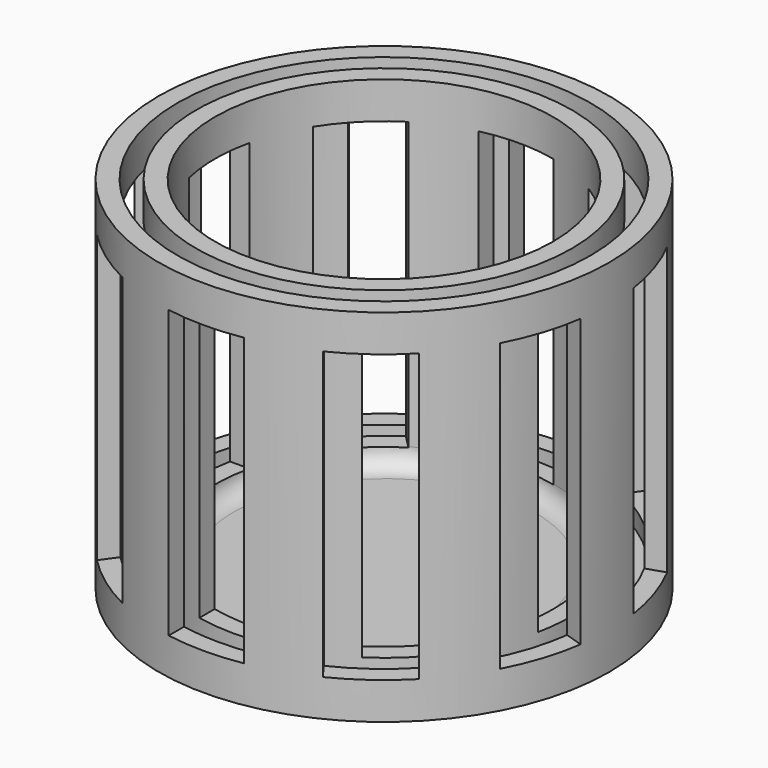
from build123d import *

# Parameters (mm, degrees)
F2_W            = 20
F2_H            = 76.3443418741
F3_REACH        = 138.9215837294
F3_COPIES_COUNT = 8
F5_W            = 20
F5_H            = 76.3443418741
F6_REACH        = 213.9215837294
F6_COPIES_COUNT = 10


# Not quite as in the source:
# - a pattern or mirror of a feature is missing from the dataset's text; its kind, count and spacing are read off the source's solid


with BuildPart() as f1:
    # F0 (on Front) → F1 (revolve)
    with BuildSketch(Plane.XZ):
        with BuildLine():
            Line((0, 5), (0, 0))
            Line((0, 0), (60, 0))
            Line((60, 0), (60, 96))
            Line((60, 96), (55, 96))
            Line((55, 96), (55, 5))
            Line((55, 5), (50, 5))
            Line((50, 5), (50, 96))
            Line((50, 96), (45, 96))
            Line((45, 96), (45, 10))
            ThreePointArc((45, 10), (43.5355339059, 6.4644660941), (40, 5))
            Line((40, 5), (0, 5))
        make_face()
    revolve(axis=Axis((0, 0, 2.5), (0, 0, 1)))

    f3_end = f1.faces().sort_by_distance((-50, 0, 50.5))[0]
    # F2 (on Front) → F3 (cut, up to a face of the model that its end follows)
    with BuildSketch(Plane.XZ):
        with Locations((0, 48)):
            Rectangle(F2_W, F2_H)
    f3_long = extrude(amount=F3_REACH, mode=Mode.PRIVATE)
    f3 = split(f3_long, bisect_by=f3_end, keep=Keep.BOTTOM, mode=Mode.PRIVATE)
    add(f3, mode=Mode.SUBTRACT)

    # F3_copies: F3 ×8 about axis
    f3_copies_axis = Axis((0, 0, 0), (0, 0, 1))
    for i in range(1, F3_COPIES_COUNT):
        add(f3.rotate(f3_copies_axis, i * 360 / F3_COPIES_COUNT), mode=Mode.SUBTRACT)

    f6_end = f1.faces().sort_by_distance((-55, 0, 50.5))[0]
    # F5 (on offset) → F6 (cut, up to a face of the model that its end follows)
    with BuildSketch(Plane.XZ.offset(75)):
        with Locations((0, 48)):
            Rectangle(F5_W, F5_H)
    f6_long = extrude(amount=-F6_REACH, mode=Mode.PRIVATE)
    f6 = split(f6_long, bisect_by=f6_end, keep=Keep.ALL, mode=Mode.PRIVATE).solids().sort_by_distance((0, -75, 48))[0]
    add(f6, mode=Mode.SUBTRACT)

    # F6_copies: F6 ×10 about axis
    f6_copies_axis = Axis((0, 0, 0), (0, 0, 1))
    for i in range(1, F6_COPIES_COUNT):
        add(f6.rotate(f6_copies_axis, i * 360 / F6_COPIES_COUNT), mode=Mode.SUBTRACT)


solid = f1.part
